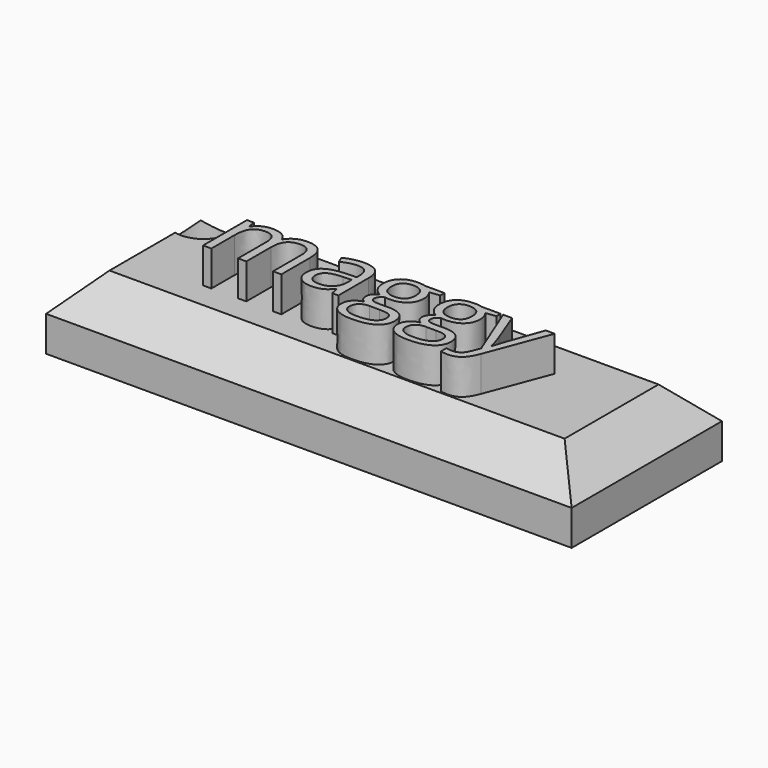
from build123d import *

# Parameters (mm, degrees)
F1_DEPTH     = 5.08
F0_W         = 37.9114933312
F0_H         = 13.5506950319
F0_R         = 2.0596348117
F0_TEXT_SIZE = 7.4012877627
F2_DEPTH     = 7.62
F3_T1_DEPTH  = 26.6148446107
F3_T3_DEPTH  = 50.9756429101


# Not quite as in the source:
# - a fillet or chamfer that OpenCascade refuses, or shapes differently, is made with other operations: its cross-section is extruded or revolved along the edge and cut away or added
# - Text() gives the source's letters only with a copy of the font that has no kerning and outlines rounded to 1/6400 em; it was checked with that copy


with BuildPart() as f1:
    # F0 (on Top) → F1 (new body)
    with BuildSketch(Plane.XY):
        with BuildLine():
            add(Edge.make_bspline(
                [(-45.2039994966, 35.4939687309), (-45.4318203855, 35.2667260676), (-45.4318203855, 34.818022997)],
                knots=[0, 0, 0, 1, 1, 1], degree=2))
            add(Edge.make_bspline(
                [(-45.4318203855, 34.818022997), (-45.4318203855, 34.4028570115), (-45.1970607893, 34.1894917627)],
                knots=[0, 0, 0, 1, 1, 1], degree=2))
            add(Edge.make_bspline(
                [(-45.1970607893, 34.1894917627), (-44.9623011931, 33.976126514), (-44.5425094028, 33.976126514)],
                knots=[0, 0, 0, 1, 1, 1], degree=2))
            add(Edge.make_bspline(
                [(-44.5425094028, 33.976126514), (-43.6647629322, 33.976126514), (-43.6647629322, 34.8295875091)],
                knots=[0, 0, 0, 1, 1, 1], degree=2))
            add(Edge.make_bspline(
                [(-43.6647629322, 34.8295875091), (-43.6647629322, 35.7212113942), (-44.5529174637, 35.7212113942)],
                knots=[0, 0, 0, 1, 1, 1], degree=2))
            add(Edge.make_bspline(
                [(-44.5529174637, 35.7212113942), (-44.9761786076, 35.7212113942), (-45.2039994966, 35.4939687309)],
                knots=[0, 0, 0, 1, 1, 1], degree=2))
        make_face()
    extrude(amount=F1_DEPTH)


with BuildPart() as f1b:
    # F0 (on Top) → F1, piece 2 (new body)
    with BuildSketch(Plane.XY):
        with BuildLine():
            add(Edge.make_bspline(
                [(-41.1494815441, 35.4939687309), (-41.377302433, 35.2667260676), (-41.377302433, 34.818022997)],
                knots=[0, 0, 0, 1, 1, 1], degree=2))
            add(Edge.make_bspline(
                [(-41.377302433, 34.818022997), (-41.377302433, 34.4028570115), (-41.1425428368, 34.1894917627)],
                knots=[0, 0, 0, 1, 1, 1], degree=2))
            add(Edge.make_bspline(
                [(-41.1425428368, 34.1894917627), (-40.9077832406, 33.976126514), (-40.4879914503, 33.976126514)],
                knots=[0, 0, 0, 1, 1, 1], degree=2))
            add(Edge.make_bspline(
                [(-40.4879914503, 33.976126514), (-39.6102449797, 33.976126514), (-39.6102449797, 34.8295875091)],
                knots=[0, 0, 0, 1, 1, 1], degree=2))
            add(Edge.make_bspline(
                [(-39.6102449797, 34.8295875091), (-39.6102449797, 35.7212113942), (-40.4983995112, 35.7212113942)],
                knots=[0, 0, 0, 1, 1, 1], degree=2))
            add(Edge.make_bspline(
                [(-40.4983995112, 35.7212113942), (-40.9216606551, 35.7212113942), (-41.1494815441, 35.4939687309)],
                knots=[0, 0, 0, 1, 1, 1], degree=2))
        make_face()
    extrude(amount=F1_DEPTH)


with BuildPart() as f1c:
    # F0 (on Top) → F1, piece 3 (new body)
    with BuildSketch(Plane.XY):
        with BuildLine():
            add(Edge.make_bspline(
                [(-41.4744443349, 32.0211457385), (-41.7022652239, 31.8262837092), (-41.7022652239, 31.4608451259)],
                knots=[0, 0, 0, 1, 1, 1], degree=2))
            add(Edge.make_bspline(
                [(-41.7022652239, 31.4608451259), (-41.7022652239, 31.1393516887), (-41.4310774144, 30.972822714)],
                knots=[0, 0, 0, 1, 1, 1], degree=2))
            add(Edge.make_bspline(
                [(-41.4310774144, 30.972822714), (-41.159889605, 30.8062937394), (-40.6545204249, 30.8062937394)],
                knots=[0, 0, 0, 1, 1, 1], degree=2))
            add(Edge.make_bspline(
                [(-40.6545204249, 30.8062937394), (-39.8993577829, 30.8062937394), (-39.5362321021, 31.0323799515)],
                knots=[0, 0, 0, 1, 1, 1], degree=2))
            add(Edge.make_bspline(
                [(-39.5362321021, 31.0323799515), (-39.1731064212, 31.2584661636), (-39.1731064212, 31.6447208687)],
                knots=[0, 0, 0, 1, 1, 1], degree=2))
            add(Edge.make_bspline(
                [(-39.1731064212, 31.6447208687), (-39.1731064212, 31.9662143059), (-39.3714378042, 32.0911110369)],
                knots=[0, 0, 0, 1, 1, 1], degree=2))
            add(Edge.make_bspline(
                [(-39.3714378042, 32.0911110369), (-39.5697691872, 32.2160077679), (-40.1190835134, 32.2160077679)],
                knots=[0, 0, 0, 1, 1, 1], degree=2))
            Line((-40.1190835134, 32.2160077679), (-40.8383961678, 32.2160077679))
            add(Edge.make_bspline(
                [(-40.8383961678, 32.2160077679), (-41.246623446, 32.2160077679), (-41.4744443349, 32.0211457385)],
                knots=[0, 0, 0, 1, 1, 1], degree=2))
        make_face()
    extrude(amount=F1_DEPTH)


with BuildPart() as f1d:
    # F0 (on Top) → F1, piece 4 (new body)
    with BuildSketch(Plane.XY):
        with BuildLine():
            add(Edge.make_bspline(
                [(-45.5289622874, 32.0211457385), (-45.7567831763, 31.8262837092), (-45.7567831763, 31.4608451259)],
                knots=[0, 0, 0, 1, 1, 1], degree=2))
            add(Edge.make_bspline(
                [(-45.7567831763, 31.4608451259), (-45.7567831763, 31.1393516887), (-45.4855953669, 30.972822714)],
                knots=[0, 0, 0, 1, 1, 1], degree=2))
            add(Edge.make_bspline(
                [(-45.4855953669, 30.972822714), (-45.2144075575, 30.8062937394), (-44.7090383774, 30.8062937394)],
                knots=[0, 0, 0, 1, 1, 1], degree=2))
            add(Edge.make_bspline(
                [(-44.7090383774, 30.8062937394), (-43.9538757354, 30.8062937394), (-43.5907500545, 31.0323799515)],
                knots=[0, 0, 0, 1, 1, 1], degree=2))
            add(Edge.make_bspline(
                [(-43.5907500545, 31.0323799515), (-43.2276243737, 31.2584661636), (-43.2276243737, 31.6447208687)],
                knots=[0, 0, 0, 1, 1, 1], degree=2))
            add(Edge.make_bspline(
                [(-43.2276243737, 31.6447208687), (-43.2276243737, 31.9662143059), (-43.4259557567, 32.0911110369)],
                knots=[0, 0, 0, 1, 1, 1], degree=2))
            add(Edge.make_bspline(
                [(-43.4259557567, 32.0911110369), (-43.6242871397, 32.2160077679), (-44.1736014658, 32.2160077679)],
                knots=[0, 0, 0, 1, 1, 1], degree=2))
            Line((-44.1736014658, 32.2160077679), (-44.8929141203, 32.2160077679))
            add(Edge.make_bspline(
                [(-44.8929141203, 32.2160077679), (-45.3011413984, 32.2160077679), (-45.5289622874, 32.0211457385)],
                knots=[0, 0, 0, 1, 1, 1], degree=2))
        make_face()
    extrude(amount=F1_DEPTH)


with BuildPart() as f1e:
    # F0 (on Top) → F1, piece 5 (new body)
    with BuildSketch(Plane.XY):
        with BuildLine():
            add(Edge.make_bspline(
                [(-49.4262028749, 32.7184858199), (-49.2296061687, 32.5490657172), (-48.8757320976, 32.5490657172)],
                knots=[0, 0, 0, 1, 1, 1], degree=2))
            add(Edge.make_bspline(
                [(-48.8757320976, 32.5490657172), (-48.3148532593, 32.5490657172), (-47.9950944989, 32.8561035143)],
                knots=[0, 0, 0, 1, 1, 1], degree=2))
            add(Edge.make_bspline(
                [(-47.9950944989, 32.8561035143), (-47.6753357386, 33.1631413113), (-47.6753357386, 33.7159249911)],
                knots=[0, 0, 0, 1, 1, 1], degree=2))
            Line((-47.6753357386, 33.7159249911), (-47.6753357386, 34.0732684158))
            Line((-47.6753357386, 34.0732684158), (-48.2755339181, 34.0489829404))
            add(Edge.make_bspline(
                [(-48.2755339181, 34.0489829404), (-48.9913772189, 34.0235410137), (-49.3070884, 33.8263660819)],
                knots=[0, 0, 0, 1, 1, 1], degree=2))
            add(Edge.make_bspline(
                [(-49.3070884, 33.8263660819), (-49.6227995811, 33.6291911501), (-49.6227995811, 33.2140251647)],
                knots=[0, 0, 0, 1, 1, 1], degree=2))
            add(Edge.make_bspline(
                [(-49.6227995811, 33.2140251647), (-49.6227995811, 32.8879059226), (-49.4262028749, 32.7184858199)],
                knots=[0, 0, 0, 1, 1, 1], degree=2))
        make_face()
    extrude(amount=F1_DEPTH)


with BuildPart() as f1f:
    # F0 (on Top) → F1, piece 6 (new body)
    with BuildSketch(Plane.XY):
        with Locations((-45.6764977425, 34.4857554883)):
            Rectangle(F0_W, F0_H)
        with BuildLine():
            Line((-51.192103877, 32.1258045733), (-51.7911456053, 32.1258045733))
            Line((-51.7911456053, 32.1258045733), (-51.7911456053, 34.7023778757))
            add(Edge.make_bspline(
                [(-51.7911456053, 34.7023778757), (-51.7911456053, 35.176522873), (-51.9935245676, 35.413017146)],
                knots=[0, 0, 0, 1, 1, 1], degree=2))
            add(Edge.make_bspline(
                [(-51.9935245676, 35.413017146), (-52.1959035298, 35.649511419), (-52.6226340274, 35.649511419)],
                knots=[0, 0, 0, 1, 1, 1], degree=2))
            add(Edge.make_bspline(
                [(-52.6226340274, 35.649511419), (-53.1823564145, 35.649511419), (-53.4500748702, 35.3280179819)],
                knots=[0, 0, 0, 1, 1, 1], degree=2))
            add(Edge.make_bspline(
                [(-53.4500748702, 35.3280179819), (-53.717793326, 35.0065245447), (-53.717793326, 34.3380957436)],
                knots=[0, 0, 0, 1, 1, 1], degree=2))
            Line((-53.717793326, 34.3380957436), (-53.717793326, 32.1258045733))
            Line((-53.717793326, 32.1258045733), (-54.3179915055, 32.1258045733))
            Line((-54.3179915055, 32.1258045733), (-54.3179915055, 34.7023778757))
            add(Edge.make_bspline(
                [(-54.3179915055, 34.7023778757), (-54.3179915055, 35.176522873), (-54.5203704678, 35.413017146)],
                knots=[0, 0, 0, 1, 1, 1], degree=2))
            add(Edge.make_bspline(
                [(-54.5203704678, 35.413017146), (-54.7227494301, 35.649511419), (-55.1529492813, 35.649511419)],
                knots=[0, 0, 0, 1, 1, 1], degree=2))
            add(Edge.make_bspline(
                [(-55.1529492813, 35.649511419), (-55.716141022, 35.649511419), (-55.9780772217, 35.3118276649)],
                knots=[0, 0, 0, 1, 1, 1], degree=2))
            add(Edge.make_bspline(
                [(-55.9780772217, 35.3118276649), (-56.2400134214, 34.9741439107), (-56.2400134214, 34.2039474029)],
                knots=[0, 0, 0, 1, 1, 1], degree=2))
            Line((-56.2400134214, 34.2039474029), (-56.2400134214, 32.1258045733))
            Line((-56.2400134214, 32.1258045733), (-56.8402116009, 32.1258045733))
            Line((-56.8402116009, 32.1258045733), (-56.8402116009, 36.0866499775))
            Line((-56.8402116009, 36.0866499775), (-56.3521891891, 36.0866499775))
            Line((-56.3521891891, 36.0866499775), (-56.2550472872, 35.5442743587))
            Line((-56.2550472872, 35.5442743587), (-56.2261360068, 35.5442743587))
            add(Edge.make_bspline(
                [(-56.2261360068, 35.5442743587), (-56.0561376785, 35.8333871619), (-55.7467869791, 35.9964467829)],
                knots=[0, 0, 0, 1, 1, 1], degree=2))
            add(Edge.make_bspline(
                [(-55.7467869791, 35.9964467829), (-55.4374362796, 36.1595064039), (-55.0546509282, 36.1595064039)],
                knots=[0, 0, 0, 1, 1, 1], degree=2))
            add(Edge.make_bspline(
                [(-55.0546509282, 36.1595064039), (-54.1260206042, 36.1595064039), (-53.8403771546, 35.486451798)],
                knots=[0, 0, 0, 1, 1, 1], degree=2))
            Line((-53.8403771546, 35.486451798), (-53.8114658743, 35.486451798))
            add(Edge.make_bspline(
                [(-53.8114658743, 35.486451798), (-53.6345288387, 35.7975371743), (-53.2985797614, 35.9785217891)],
                knots=[0, 0, 0, 1, 1, 1], degree=2))
            add(Edge.make_bspline(
                [(-53.2985797614, 35.9785217891), (-52.962630684, 36.1595064039), (-52.5324308328, 36.1595064039)],
                knots=[0, 0, 0, 1, 1, 1], degree=2))
            add(Edge.make_bspline(
                [(-52.5324308328, 36.1595064039), (-51.8605326781, 36.1595064039), (-51.5263182776, 35.8143057169)],
                knots=[0, 0, 0, 1, 1, 1], degree=2))
            add(Edge.make_bspline(
                [(-51.5263182776, 35.8143057169), (-51.192103877, 35.4691050298), (-51.192103877, 34.7093165829)],
                knots=[0, 0, 0, 1, 1, 1], degree=2))
            Line((-51.192103877, 34.7093165829), (-51.192103877, 32.1258045733))
        make_face(mode=Mode.SUBTRACT)
        with BuildLine():
            Line((-47.0751375591, 32.1258045733), (-47.520371276, 32.1258045733))
            Line((-47.520371276, 32.1258045733), (-47.639485751, 32.6901527652))
            Line((-47.639485751, 32.6901527652), (-47.6683970313, 32.6901527652))
            add(Edge.make_bspline(
                [(-47.6683970313, 32.6901527652), (-47.9644485418, 32.3177754746), (-48.2587653755, 32.1853618108)],
                knots=[0, 0, 0, 1, 1, 1], degree=2))
            add(Edge.make_bspline(
                [(-48.2587653755, 32.1853618108), (-48.5530822092, 32.0529481469), (-48.9948465725, 32.0529481469)],
                knots=[0, 0, 0, 1, 1, 1], degree=2))
            add(Edge.make_bspline(
                [(-48.9948465725, 32.0529481469), (-49.5834802399, 32.0529481469), (-49.9176946404, 32.3570948159)],
                knots=[0, 0, 0, 1, 1, 1], degree=2))
            add(Edge.make_bspline(
                [(-49.9176946404, 32.3570948159), (-50.2519090409, 32.6612414849), (-50.2519090409, 33.2209638719)],
                knots=[0, 0, 0, 1, 1, 1], degree=2))
            add(Edge.make_bspline(
                [(-50.2519090409, 33.2209638719), (-50.2519090409, 34.4202037797), (-48.3333564787, 34.4780263404)],
                knots=[0, 0, 0, 1, 1, 1], degree=2))
            Line((-48.3333564787, 34.4780263404), (-47.661458324, 34.4999989134))
            Line((-47.661458324, 34.4999989134), (-47.661458324, 34.7463230218))
            add(Edge.make_bspline(
                [(-47.661458324, 34.7463230218), (-47.661458324, 35.2123728606), (-47.8615243838, 35.4344114934)],
                knots=[0, 0, 0, 1, 1, 1], degree=2))
            add(Edge.make_bspline(
                [(-47.8615243838, 35.4344114934), (-48.0615904437, 35.6564501263), (-48.503354807, 35.6564501263)],
                knots=[0, 0, 0, 1, 1, 1], degree=2))
            add(Edge.make_bspline(
                [(-48.503354807, 35.6564501263), (-48.9983159261, 35.6564501263), (-49.6227995811, 35.3534599085)],
                knots=[0, 0, 0, 1, 1, 1], degree=2))
            Line((-49.6227995811, 35.3534599085), (-49.8078317752, 35.8125710401))
            add(Edge.make_bspline(
                [(-49.8078317752, 35.8125710401), (-49.5152496183, 35.9710048562), (-49.1665795776, 36.0612080508)],
                knots=[0, 0, 0, 1, 1, 1], degree=2))
            add(Edge.make_bspline(
                [(-49.1665795776, 36.0612080508), (-48.8179095369, 36.1514112455), (-48.4663483682, 36.1514112455)],
                knots=[0, 0, 0, 1, 1, 1], degree=2))
            add(Edge.make_bspline(
                [(-48.4663483682, 36.1514112455), (-47.7586002259, 36.1514112455), (-47.4168688925, 35.8374347411)],
                knots=[0, 0, 0, 1, 1, 1], degree=2))
            add(Edge.make_bspline(
                [(-47.4168688925, 35.8374347411), (-47.0751375591, 35.5234582368), (-47.0751375591, 34.8295875091)],
                knots=[0, 0, 0, 1, 1, 1], degree=2))
            Line((-47.0751375591, 34.8295875091), (-47.0751375591, 32.1258045733))
        make_face(mode=Mode.SUBTRACT)
        with BuildLine():
            Line((-43.96775315, 36.0866499775), (-42.5985149139, 36.0866499775))
            Line((-42.5985149139, 36.0866499775), (-42.5985149139, 35.7073339797))
            Line((-42.5985149139, 35.7073339797), (-43.3317049828, 35.6206001387))
            add(Edge.make_bspline(
                [(-43.3317049828, 35.6206001387), (-43.2310937273, 35.4945469565), (-43.1512985936, 35.2898550918)],
                knots=[0, 0, 0, 1, 1, 1], degree=2))
            add(Edge.make_bspline(
                [(-43.1512985936, 35.2898550918), (-43.0715034599, 35.0851632271), (-43.0715034599, 34.8295875091)],
                knots=[0, 0, 0, 1, 1, 1], degree=2))
            add(Edge.make_bspline(
                [(-43.0715034599, 34.8295875091), (-43.0715034599, 34.2467360978), (-43.4693226772, 33.8998007339)],
                knots=[0, 0, 0, 1, 1, 1], degree=2))
            add(Edge.make_bspline(
                [(-43.4693226772, 33.8998007339), (-43.8671418944, 33.55286537), (-44.5610126222, 33.55286537)],
                knots=[0, 0, 0, 1, 1, 1], degree=2))
            add(Edge.make_bspline(
                [(-44.5610126222, 33.55286537), (-44.7379496578, 33.55286537), (-44.8929141203, 33.5817766504)],
                knots=[0, 0, 0, 1, 1, 1], degree=2))
            add(Edge.make_bspline(
                [(-44.8929141203, 33.5817766504), (-45.2756994718, 33.3793976881), (-45.2756994718, 33.0729381167)],
                knots=[0, 0, 0, 1, 1, 1], degree=2))
            add(Edge.make_bspline(
                [(-45.2756994718, 33.0729381167), (-45.2756994718, 32.9098784957), (-45.1421293567, 32.8323962644)],
                knots=[0, 0, 0, 1, 1, 1], degree=2))
            add(Edge.make_bspline(
                [(-45.1421293567, 32.8323962644), (-45.0085592416, 32.7549140331), (-44.6835964507, 32.7549140331)],
                knots=[0, 0, 0, 1, 1, 1], degree=2))
            Line((-44.6835964507, 32.7549140331), (-43.9827870157, 32.7549140331))
            add(Edge.make_bspline(
                [(-43.9827870157, 32.7549140331), (-43.3386436901, 32.7549140331), (-42.9940212287, 32.4837262237)],
                knots=[0, 0, 0, 1, 1, 1], degree=2))
            add(Edge.make_bspline(
                [(-42.9940212287, 32.4837262237), (-42.6493987672, 32.2125384143), (-42.6493987672, 31.6956047221)],
                knots=[0, 0, 0, 1, 1, 1], degree=2))
            add(Edge.make_bspline(
                [(-42.6493987672, 31.6956047221), (-42.6493987672, 31.0375839819), (-43.1767405203, 30.6923832949)],
                knots=[0, 0, 0, 1, 1, 1], degree=2))
            add(Edge.make_bspline(
                [(-43.1767405203, 30.6923832949), (-43.7040822734, 30.3471826078), (-44.7159770847, 30.3471826078)],
                knots=[0, 0, 0, 1, 1, 1], degree=2))
            add(Edge.make_bspline(
                [(-44.7159770847, 30.3471826078), (-45.4931122998, 30.3471826078), (-45.9140605413, 30.6362954111)],
                knots=[0, 0, 0, 1, 1, 1], degree=2))
            add(Edge.make_bspline(
                [(-45.9140605413, 30.6362954111), (-46.3350087828, 30.9254082143), (-46.3350087828, 31.4539064186)],
                knots=[0, 0, 0, 1, 1, 1], degree=2))
            add(Edge.make_bspline(
                [(-46.3350087828, 31.4539064186), (-46.3350087828, 31.814719197), (-46.1037185402, 32.0789682992)],
                knots=[0, 0, 0, 1, 1, 1], degree=2))
            add(Edge.make_bspline(
                [(-46.1037185402, 32.0789682992), (-45.8724282976, 32.3432174013), (-45.4537929585, 32.4368899496)],
                knots=[0, 0, 0, 1, 1, 1], degree=2))
            add(Edge.make_bspline(
                [(-45.4537929585, 32.4368899496), (-45.6052880674, 32.5051205711), (-45.7082122254, 32.6496769727)],
                knots=[0, 0, 0, 1, 1, 1], degree=2))
            add(Edge.make_bspline(
                [(-45.7082122254, 32.6496769727), (-45.8111363833, 32.7942333744), (-45.8111363833, 32.9862042757)],
                knots=[0, 0, 0, 1, 1, 1], degree=2))
            add(Edge.make_bspline(
                [(-45.8111363833, 32.9862042757), (-45.8111363833, 33.2024606525), (-45.695491262, 33.3655202735)],
                knots=[0, 0, 0, 1, 1, 1], degree=2))
            add(Edge.make_bspline(
                [(-45.695491262, 33.3655202735), (-45.5798461408, 33.5285798946), (-45.3300526788, 33.6800750035)],
                knots=[0, 0, 0, 1, 1, 1], degree=2))
            add(Edge.make_bspline(
                [(-45.3300526788, 33.6800750035), (-45.6376687014, 33.8061281857), (-45.830796054, 34.1096966291)],
                knots=[0, 0, 0, 1, 1, 1], degree=2))
            add(Edge.make_bspline(
                [(-45.830796054, 34.1096966291), (-46.0239234065, 34.4132650724), (-46.0239234065, 34.8041455824)],
                knots=[0, 0, 0, 1, 1, 1], degree=2))
            add(Edge.make_bspline(
                [(-46.0239234065, 34.8041455824), (-46.0239234065, 35.4540711641), (-45.6336211222, 35.806788784)],
                knots=[0, 0, 0, 1, 1, 1], degree=2))
            add(Edge.make_bspline(
                [(-45.6336211222, 35.806788784), (-45.2433188378, 36.1595064039), (-44.5286319882, 36.1595064039)],
                knots=[0, 0, 0, 1, 1, 1], degree=2))
            add(Edge.make_bspline(
                [(-44.5286319882, 36.1595064039), (-44.2175466119, 36.1595064039), (-43.96775315, 36.0866499775)],
                knots=[0, 0, 0, 1, 1, 1], degree=2))
        make_face(mode=Mode.SUBTRACT)
        with BuildLine():
            Line((-39.9132351975, 36.0866499775), (-38.5439969614, 36.0866499775))
            Line((-38.5439969614, 36.0866499775), (-38.5439969614, 35.7073339797))
            Line((-38.5439969614, 35.7073339797), (-39.2771870304, 35.6206001387))
            add(Edge.make_bspline(
                [(-39.2771870304, 35.6206001387), (-39.1765757748, 35.4945469565), (-39.0967806412, 35.2898550918)],
                knots=[0, 0, 0, 1, 1, 1], degree=2))
            add(Edge.make_bspline(
                [(-39.0967806412, 35.2898550918), (-39.0169855075, 35.0851632271), (-39.0169855075, 34.8295875091)],
                knots=[0, 0, 0, 1, 1, 1], degree=2))
            add(Edge.make_bspline(
                [(-39.0169855075, 34.8295875091), (-39.0169855075, 34.2467360978), (-39.4148047247, 33.8998007339)],
                knots=[0, 0, 0, 1, 1, 1], degree=2))
            add(Edge.make_bspline(
                [(-39.4148047247, 33.8998007339), (-39.8126239419, 33.55286537), (-40.5064946697, 33.55286537)],
                knots=[0, 0, 0, 1, 1, 1], degree=2))
            add(Edge.make_bspline(
                [(-40.5064946697, 33.55286537), (-40.6834317053, 33.55286537), (-40.8383961678, 33.5817766504)],
                knots=[0, 0, 0, 1, 1, 1], degree=2))
            add(Edge.make_bspline(
                [(-40.8383961678, 33.5817766504), (-41.2211815193, 33.3793976881), (-41.2211815193, 33.0729381167)],
                knots=[0, 0, 0, 1, 1, 1], degree=2))
            add(Edge.make_bspline(
                [(-41.2211815193, 33.0729381167), (-41.2211815193, 32.9098784957), (-41.0876114042, 32.8323962644)],
                knots=[0, 0, 0, 1, 1, 1], degree=2))
            add(Edge.make_bspline(
                [(-41.0876114042, 32.8323962644), (-40.9540412891, 32.7549140331), (-40.6290784983, 32.7549140331)],
                knots=[0, 0, 0, 1, 1, 1], degree=2))
            Line((-40.6290784983, 32.7549140331), (-39.9282690632, 32.7549140331))
            add(Edge.make_bspline(
                [(-39.9282690632, 32.7549140331), (-39.2841257376, 32.7549140331), (-38.9395032762, 32.4837262237)],
                knots=[0, 0, 0, 1, 1, 1], degree=2))
            add(Edge.make_bspline(
                [(-38.9395032762, 32.4837262237), (-38.5948808147, 32.2125384143), (-38.5948808147, 31.6956047221)],
                knots=[0, 0, 0, 1, 1, 1], degree=2))
            add(Edge.make_bspline(
                [(-38.5948808147, 31.6956047221), (-38.5948808147, 31.0375839819), (-39.1222225678, 30.6923832949)],
                knots=[0, 0, 0, 1, 1, 1], degree=2))
            add(Edge.make_bspline(
                [(-39.1222225678, 30.6923832949), (-39.6495643209, 30.3471826078), (-40.6614591322, 30.3471826078)],
                knots=[0, 0, 0, 1, 1, 1], degree=2))
            add(Edge.make_bspline(
                [(-40.6614591322, 30.3471826078), (-41.4385943473, 30.3471826078), (-41.8595425888, 30.6362954111)],
                knots=[0, 0, 0, 1, 1, 1], degree=2))
            add(Edge.make_bspline(
                [(-41.8595425888, 30.6362954111), (-42.2804908303, 30.9254082143), (-42.2804908303, 31.4539064186)],
                knots=[0, 0, 0, 1, 1, 1], degree=2))
            add(Edge.make_bspline(
                [(-42.2804908303, 31.4539064186), (-42.2804908303, 31.814719197), (-42.0492005877, 32.0789682992)],
                knots=[0, 0, 0, 1, 1, 1], degree=2))
            add(Edge.make_bspline(
                [(-42.0492005877, 32.0789682992), (-41.8179103451, 32.3432174013), (-41.3992750061, 32.4368899496)],
                knots=[0, 0, 0, 1, 1, 1], degree=2))
            add(Edge.make_bspline(
                [(-41.3992750061, 32.4368899496), (-41.550770115, 32.5051205711), (-41.6536942729, 32.6496769727)],
                knots=[0, 0, 0, 1, 1, 1], degree=2))
            add(Edge.make_bspline(
                [(-41.6536942729, 32.6496769727), (-41.7566184309, 32.7942333744), (-41.7566184309, 32.9862042757)],
                knots=[0, 0, 0, 1, 1, 1], degree=2))
            add(Edge.make_bspline(
                [(-41.7566184309, 32.9862042757), (-41.7566184309, 33.2024606525), (-41.6409733096, 33.3655202735)],
                knots=[0, 0, 0, 1, 1, 1], degree=2))
            add(Edge.make_bspline(
                [(-41.6409733096, 33.3655202735), (-41.5253281883, 33.5285798946), (-41.2755347263, 33.6800750035)],
                knots=[0, 0, 0, 1, 1, 1], degree=2))
            add(Edge.make_bspline(
                [(-41.2755347263, 33.6800750035), (-41.5831507489, 33.8061281857), (-41.7762781015, 34.1096966291)],
                knots=[0, 0, 0, 1, 1, 1], degree=2))
            add(Edge.make_bspline(
                [(-41.7762781015, 34.1096966291), (-41.969405454, 34.4132650724), (-41.969405454, 34.8041455824)],
                knots=[0, 0, 0, 1, 1, 1], degree=2))
            add(Edge.make_bspline(
                [(-41.969405454, 34.8041455824), (-41.969405454, 35.4540711641), (-41.5791031697, 35.806788784)],
                knots=[0, 0, 0, 1, 1, 1], degree=2))
            add(Edge.make_bspline(
                [(-41.5791031697, 35.806788784), (-41.1888008853, 36.1595064039), (-40.4741140357, 36.1595064039)],
                knots=[0, 0, 0, 1, 1, 1], degree=2))
            add(Edge.make_bspline(
                [(-40.4741140357, 36.1595064039), (-40.1630286595, 36.1595064039), (-39.9132351975, 36.0866499775)],
                knots=[0, 0, 0, 1, 1, 1], degree=2))
        make_face(mode=Mode.SUBTRACT)
        with BuildLine():
            Line((-36.7619056423, 32.1038320003), (-38.3601212185, 36.0866499775))
            Line((-38.3601212185, 36.0866499775), (-37.7159778929, 36.0866499775))
            Line((-37.7159778929, 36.0866499775), (-36.8486394832, 33.8281007587))
            add(Edge.make_bspline(
                [(-36.8486394832, 33.8281007587), (-36.5641524849, 33.0544348973), (-36.4947654121, 32.710968887)],
                knots=[0, 0, 0, 1, 1, 1], degree=2))
            Line((-36.4947654121, 32.710968887), (-36.4658541318, 32.710968887))
            add(Edge.make_bspline(
                [(-36.4658541318, 32.710968887), (-36.4195960833, 32.8960010811), (-36.2692574256, 33.3423912493)],
                knots=[0, 0, 0, 1, 1, 1], degree=2))
            add(Edge.make_bspline(
                [(-36.2692574256, 33.3423912493), (-36.1189187679, 33.7887814175), (-35.2874303458, 36.0866499775)],
                knots=[0, 0, 0, 1, 1, 1], degree=2))
            Line((-35.2874303458, 36.0866499775), (-34.6444434714, 36.0866499775))
            Line((-34.6444434714, 36.0866499775), (-36.3467396568, 31.5764902472))
            add(Edge.make_bspline(
                [(-36.3467396568, 31.5764902472), (-36.6000024725, 30.9080614461), (-36.9376862266, 30.627622027)],
                knots=[0, 0, 0, 1, 1, 1], degree=2))
            add(Edge.make_bspline(
                [(-36.9376862266, 30.627622027), (-37.2753699808, 30.3471826078), (-37.7668617463, 30.3471826078)],
                knots=[0, 0, 0, 1, 1, 1], degree=2))
            add(Edge.make_bspline(
                [(-37.7668617463, 30.3471826078), (-38.042097135, 30.3471826078), (-38.3092373652, 30.4096309733)],
                knots=[0, 0, 0, 1, 1, 1], degree=2))
            Line((-38.3092373652, 30.4096309733), (-38.3092373652, 30.8895582267))
            add(Edge.make_bspline(
                [(-38.3092373652, 30.8895582267), (-38.1103277565, 30.8467695318), (-37.8651600994, 30.8467695318)],
                knots=[0, 0, 0, 1, 1, 1], degree=2))
            add(Edge.make_bspline(
                [(-37.8651600994, 30.8467695318), (-37.2464587005, 30.8467695318), (-36.9827878239, 31.5406402596)],
                knots=[0, 0, 0, 1, 1, 1], degree=2))
            Line((-36.9827878239, 31.5406402596), (-36.7619056423, 32.1038320003))
        make_face(mode=Mode.SUBTRACT)
        with Locations((-61.6359785199, 38.1766706705)):
            Circle(F0_R, mode=Mode.SUBTRACT)
    extrude(amount=F1_DEPTH)

    # F3: chamfer of 2.54 on 4 edges, made by hand

    # F3_s2 → F3_t1 (cut)
    with BuildSketch(Plane.XZ.offset(-47.7931777937)):
        Polygon((-26.7207510769, 2.54), (-29.2607510769, 5.08), (-26.7207510769, 5.08), align=None)
        Polygon((-64.6322444081, 2.54), (-62.0922444081, 5.08), (-64.6322444081, 5.08), align=None)
    extrude(amount=F3_T1_DEPTH, mode=Mode.SUBTRACT)

    # F3_s4 → F3_t3 (cut)
    with BuildSketch(Plane.YZ.offset(-71.1643191976)):
        Polygon((27.7104079723, 2.54), (30.2504079723, 5.08), (27.7104079723, 5.08), align=None)
        Polygon((41.2611030042, 2.54), (38.7211030042, 5.08), (41.2611030042, 5.08), align=None)
    extrude(amount=F3_T3_DEPTH, mode=Mode.SUBTRACT)


with BuildPart() as f2:
    # F0 (on Top) → F2 (new body)
    with BuildSketch(Plane.XY):
        with Locations((-57.476259768, 32.1258045733)):
            Text('maggy', F0_TEXT_SIZE, font='Open Sans', text_align=(TextAlign.LEFT, TextAlign.BOTTOM))
    extrude(amount=F2_DEPTH)


solid = Compound([f1.part, f1b.part, f1c.part, f1d.part, f1e.part, f1f.part, f2.part])
